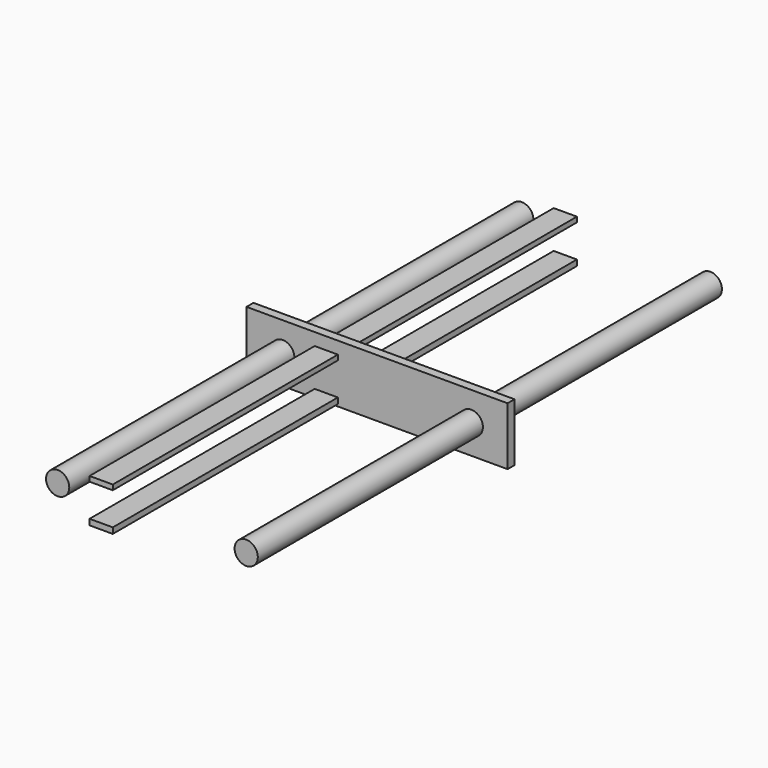
from build123d import *

# Parameters (mm, degrees)
F0_R     = 4
F1_DEPTH = 100
F0_W     = 8
F0_H     = 1.75
F0_H_2   = 2
F2_W     = 90
F2_H     = 20
F2_R     = 4
F3_DEPTH = 3
F4_W     = 8
F4_H     = 1.75
F4_H_2   = 2
F5_DEPTH = 25


with BuildPart() as f1:
    # F0 (on Front) → F1 (new body, symmetric)
    with BuildSketch(Plane.XZ):
        with Locations((-32.5, 0)):
            Circle(F0_R)
    extrude(amount=F1_DEPTH, both=True)


with BuildPart() as f1b:
    # F0 (on Front) → F1, piece 2 (new body, symmetric)
    with BuildSketch(Plane.XZ):
        with Locations((-17.5, 4.875)):
            Rectangle(F0_W, F0_H)
    extrude(amount=F1_DEPTH, both=True)


with BuildPart() as f1c:
    # F0 (on Front) → F1, piece 3 (new body, symmetric)
    with BuildSketch(Plane.XZ):
        with Locations((-17.5, -8.25)):
            Rectangle(F0_W, F0_H_2)
    extrude(amount=F1_DEPTH, both=True)


with BuildPart() as f1d:
    # F0 (on Front) → F1, piece 4 (new body, symmetric)
    with BuildSketch(Plane.XZ):
        with Locations((32.5, 0)):
            Circle(F0_R)
    extrude(amount=F1_DEPTH, both=True)


with BuildPart() as f3:
    # F2 (on Front) → F3 (new body)
    with BuildSketch(Plane.XZ):
        Rectangle(F2_W, F2_H)
        with Locations((-32.5, 0)):
            Circle(F2_R, mode=Mode.SUBTRACT)
        with Locations((32.5, 0)):
            Circle(F2_R, mode=Mode.SUBTRACT)
    extrude(amount=F3_DEPTH)

    # F4 (on face) → F5 (cut)
    with BuildSketch(Plane.XZ.offset(3)):
        with Locations((-17.5, 4.875)):
            Rectangle(F4_W, F4_H)
        with Locations((-17.5, -8.25)):
            Rectangle(F4_W, F4_H_2)
    extrude(amount=-F5_DEPTH, mode=Mode.SUBTRACT)


solid = Compound([f1.part, f1b.part, f1c.part, f1d.part, f3.part])
